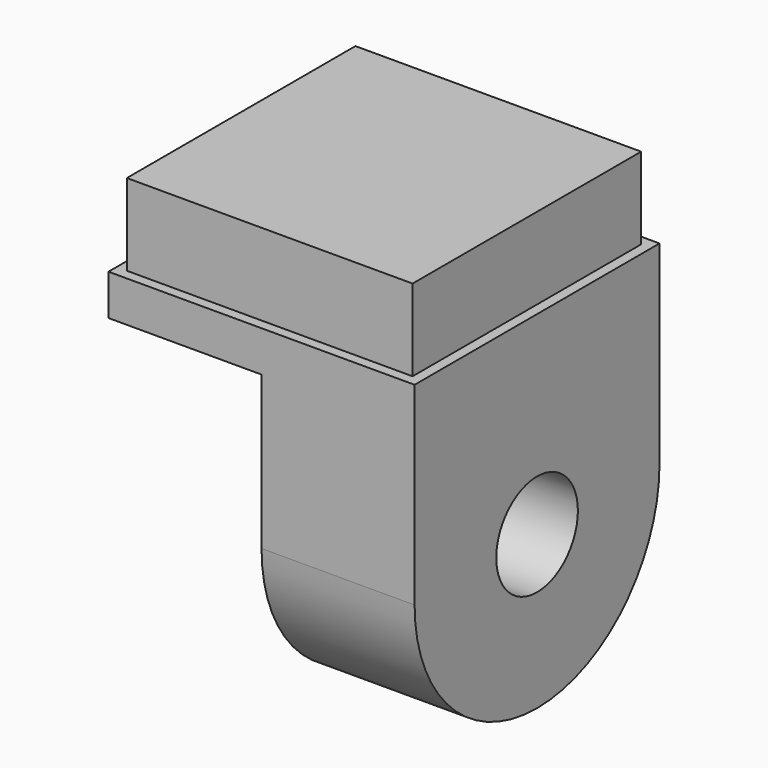
from build123d import *

# Parameters (mm, degrees)
F0_W     = 15
F0_H     = 15
F0_W_2   = 14
F0_H_2   = 14
F1_DEPTH = 2
F2_DEPTH = 6
F3_W     = 7.5
F3_H     = 15
F4_DEPTH = 15
F5_R     = 7.49999
F6_R     = 2.5
F7_DEPTH = 25


# Not quite as in the source:
# - a fillet or chamfer is up to 0.001 mm smaller than in the source, because OpenCascade refuses the exact size


with BuildPart() as f1:
    # F0 (on Top) → F1 (new body)
    with BuildSketch(Plane.XY):
        Rectangle(F0_W, F0_H)
        Rectangle(F0_W_2, F0_H_2, mode=Mode.SUBTRACT)
    extrude(amount=F1_DEPTH)

    # F0 (on Top) → F2 (join)
    with BuildSketch(Plane.XY):
        Rectangle(F0_W_2, F0_H_2)
    extrude(amount=F2_DEPTH)

    # F3 (on face) → F4 (join)
    with BuildSketch(Plane(origin=(0, 0, 0), x_dir=(1, 0, 0), z_dir=(0, 0, -1))):
        with Locations((3.75, 0)):
            Rectangle(F3_W, F3_H)
    extrude(amount=F4_DEPTH)

    # F5 (radius 7.5 in the source; OpenCascade refuses exactly that, so slightly less here)
    f5_edges = [f1.edges().sort_by_distance(p)[0] for p in [
        (3.75, 7.5, -15),
        (3.75, -7.5, -15),
    ]]
    fillet(f5_edges, radius=F5_R)

    # F6 (on face) → F7 (cut)
    with BuildSketch(Plane.YZ.offset(7.5)):
        with Locations((0, -7.5)):
            Circle(F6_R)
    extrude(amount=-F7_DEPTH, mode=Mode.SUBTRACT)


solid = f1.part
